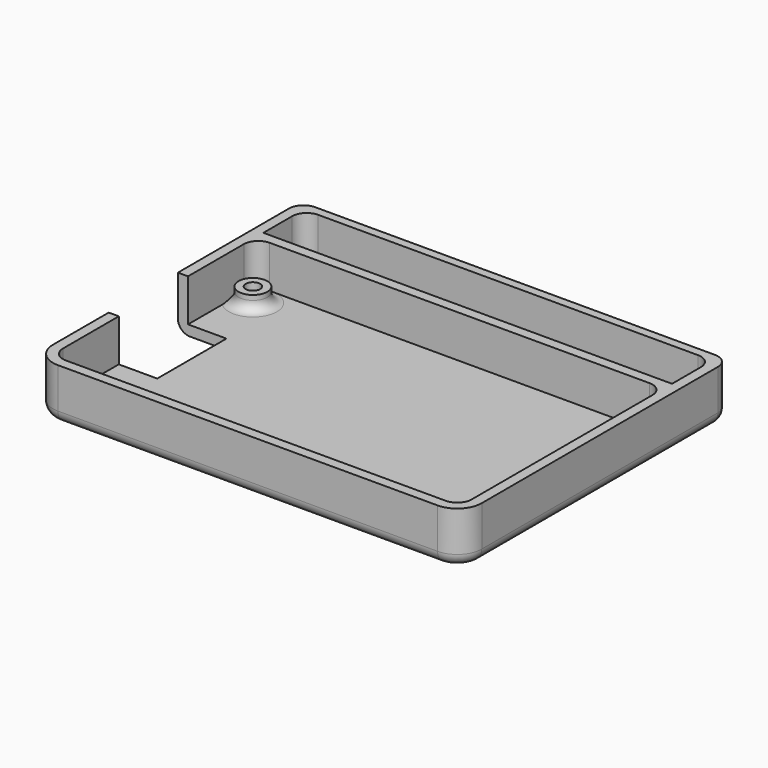
from build123d import *

# Parameters (mm, degrees)
F0_R         = 3
F0_R_2       = 1.5
F1_DEPTH     = 2.1
F2_DEPTH     = 10.9
F3_T1_DEPTH  = 61.4
F3_T3_DEPTH  = 83.2
F3_T5_DEPTH  = 35.15
F3_T7_DEPTH  = 20.75
F3_T9_DEPTH  = 79
F3_T12_ANGLE = 90
F3_T14_ANGLE = 90
F3_T16_ANGLE = 90
F3_T18_ANGLE = 90
F4_DEPTH     = 5.1


# Not quite as in the source:
# - a fillet or chamfer that OpenCascade refuses, or shapes differently, is made with other operations: its cross-section is extruded or revolved along the edge and cut away or added


with BuildPart() as f1:
    # F0 (on Top) → F1 (new body)
    with BuildSketch(Plane.XY):
        Polygon((34.5, 26.5), (-34.5, 26.5), (-34.5, 9), (-34.5, -9), (-34.5, -26.5), (34.5, -26.5), align=None)
        with BuildLine():
            add(Edge.make_bspline(
                [(-39.5, 28.6), (-36.7176169559, 28.6), (-36.7176169559, 33.85), (-36.7176169559, 39.1), (-39.5, 39.1)],
                knots=[3.1415926536, 3.1415926536, 3.1415926536, 4.7123889804, 4.7123889804, 6.2831853072, 6.2831853072, 6.2831853072], degree=2, weights=[1, 0.7071067812, 1, 0.7071067812, 1]))
            Line((-39.5, 28.6), (39.5, 28.6))
            Line((39.5, 28.6), (42.5, 28.6))
            Line((42.5, 28.6), (42.5, 36.1))
            ThreePointArc((42.5, 36.1), (41.6213203436, 38.2213203436), (39.5, 39.1))
            Line((39.5, 39.1), (0, 39.1))
            Line((0, 39.1), (-39.5, 39.1))
        make_face()
        with BuildLine():
            Line((-42.5, 9), (-42.5, 23.5))
            Line((-42.5, 23.5), (-42.5, 28.6))
            Line((-42.5, 28.6), (-42.5, 36.1))
            ThreePointArc((-42.5, 36.1), (-41.6213203436, 38.2213203436), (-39.5, 39.1))
            Line((-39.5, 39.1), (0, 39.1))
            Line((0, 39.1), (39.5, 39.1))
            ThreePointArc((39.5, 39.1), (41.6213203436, 38.2213203436), (42.5, 36.1))
            Line((42.5, 36.1), (42.5, 28.6))
            Line((42.5, 28.6), (42.5, 23.5))
            Line((42.5, 23.5), (42.5, -23.5))
            ThreePointArc((42.5, -23.5), (41.6213203436, -25.6213203436), (39.5, -26.5))
            Line((39.5, -26.5), (34.5, -26.5))
            Line((34.5, -26.5), (-34.5, -26.5))
            Line((-34.5, -26.5), (-39.5, -26.5))
            ThreePointArc((-39.5, -26.5), (-41.6213203436, -25.6213203436), (-42.5, -23.5))
            Line((-42.5, -23.5), (-42.5, -9))
            Line((-42.5, -9), (-44.6, -9))
            Line((-44.6, -9), (-44.6, -23.5))
            ThreePointArc((-44.6, -23.5), (-43.1062445841, -27.1062445841), (-39.5, -28.6))
            Line((-39.5, -28.6), (39.5, -28.6))
            ThreePointArc((39.5, -28.6), (43.1062445841, -27.1062445841), (44.6, -23.5))
            Line((44.6, -23.5), (44.6, 23.5))
            Line((44.6, 23.5), (44.6, 37.9))
            ThreePointArc((44.6, 37.9), (43.7213203436, 40.0213203436), (41.6, 40.9))
            Line((41.6, 40.9), (0, 40.9))
            Line((0, 40.9), (-41.6, 40.9))
            ThreePointArc((-41.6, 40.9), (-43.7213203436, 40.0213203436), (-44.6, 37.9))
            Line((-44.6, 37.9), (-44.6, 23.5))
            Line((-44.6, 23.5), (-44.6, 9))
            Line((-44.6, 9), (-42.5, 9))
        make_face()
        with BuildLine():
            Line((39.5, 26.5), (34.5, 26.5))
            Line((34.5, 26.5), (34.5, -26.5))
            Line((34.5, -26.5), (39.5, -26.5))
            ThreePointArc((39.5, -26.5), (41.6213203436, -25.6213203436), (42.5, -23.5))
            Line((42.5, -23.5), (42.5, 23.5))
            ThreePointArc((42.5, 23.5), (41.6213203436, 25.6213203436), (39.5, 26.5))
        make_face()
        with Locations((39, -21.5)):
            Circle(F0_R, mode=Mode.SUBTRACT)
        with Locations((39, 21.5)):
            Circle(F0_R, mode=Mode.SUBTRACT)
        with BuildLine():
            ThreePointArc((-42.5, 23.5), (-41.6213203436, 25.6213203436), (-39.5, 26.5))
            Line((-39.5, 26.5), (-34.5, 26.5))
            Line((-34.5, 26.5), (34.5, 26.5))
            Line((34.5, 26.5), (39.5, 26.5))
            ThreePointArc((39.5, 26.5), (41.6213203436, 25.6213203436), (42.5, 23.5))
            Line((42.5, 23.5), (42.5, 28.6))
            Line((42.5, 28.6), (39.5, 28.6))
            Line((39.5, 28.6), (-39.5, 28.6))
            Line((-39.5, 28.6), (-42.5, 28.6))
            Line((-42.5, 28.6), (-42.5, 23.5))
        make_face()
        with BuildLine():
            Line((-34.5, 26.5), (-39.5, 26.5))
            ThreePointArc((-39.5, 26.5), (-41.6213203436, 25.6213203436), (-42.5, 23.5))
            Line((-42.5, 23.5), (-42.5, 9))
            Line((-42.5, 9), (-34.5, 9))
            Line((-34.5, 9), (-34.5, 26.5))
        make_face()
        with Locations((-39, 21.5)):
            Circle(F0_R, mode=Mode.SUBTRACT)
        with BuildLine():
            Line((-34.5, -26.5), (-34.5, -9))
            Line((-34.5, -9), (-42.5, -9))
            Line((-42.5, -9), (-42.5, -23.5))
            ThreePointArc((-42.5, -23.5), (-41.6213203436, -25.6213203436), (-39.5, -26.5))
            Line((-39.5, -26.5), (-34.5, -26.5))
        make_face()
        with Locations((-39, -21.5)):
            Circle(F0_R, mode=Mode.SUBTRACT)
        with Locations((-39, 21.5)):
            Circle(F0_R)
        with Locations((-39, 21.5)):
            Circle(F0_R_2, mode=Mode.SUBTRACT)
        with Locations((-39, -21.5)):
            Circle(F0_R)
        with Locations((-39, -21.5)):
            Circle(F0_R_2, mode=Mode.SUBTRACT)
        with Locations((39, 21.5)):
            Circle(F0_R)
        with Locations((39, 21.5)):
            Circle(F0_R_2, mode=Mode.SUBTRACT)
        with Locations((39, -21.5)):
            Circle(F0_R)
        with Locations((39, -21.5)):
            Circle(F0_R_2, mode=Mode.SUBTRACT)
        with BuildLine():
            Line((-42.5, 36.1), (-42.5, 28.6))
            Line((-42.5, 28.6), (-39.5, 28.6))
            add(Edge.make_bspline(
                [(-39.5, 39.1), (-42.2823830441, 39.1), (-42.2823830441, 33.85), (-42.2823830441, 28.6), (-39.5, 28.6)],
                knots=[0, 0, 0, 1.5707963268, 1.5707963268, 3.1415926536, 3.1415926536, 3.1415926536], degree=2, weights=[1, 0.7071067812, 1, 0.7071067812, 1]))
            ThreePointArc((-39.5, 39.1), (-41.6213203436, 38.2213203436), (-42.5, 36.1))
        make_face()
    extrude(amount=F1_DEPTH)

    # F0 (on Top) → F2 (join)
    with BuildSketch(Plane.XY):
        with BuildLine():
            Line((-42.5, 9), (-42.5, 23.5))
            Line((-42.5, 23.5), (-42.5, 28.6))
            Line((-42.5, 28.6), (-42.5, 36.1))
            ThreePointArc((-42.5, 36.1), (-41.6213203436, 38.2213203436), (-39.5, 39.1))
            Line((-39.5, 39.1), (0, 39.1))
            Line((0, 39.1), (39.5, 39.1))
            ThreePointArc((39.5, 39.1), (41.6213203436, 38.2213203436), (42.5, 36.1))
            Line((42.5, 36.1), (42.5, 28.6))
            Line((42.5, 28.6), (42.5, 23.5))
            Line((42.5, 23.5), (42.5, -23.5))
            ThreePointArc((42.5, -23.5), (41.6213203436, -25.6213203436), (39.5, -26.5))
            Line((39.5, -26.5), (34.5, -26.5))
            Line((34.5, -26.5), (-34.5, -26.5))
            Line((-34.5, -26.5), (-39.5, -26.5))
            ThreePointArc((-39.5, -26.5), (-41.6213203436, -25.6213203436), (-42.5, -23.5))
            Line((-42.5, -23.5), (-42.5, -9))
            Line((-42.5, -9), (-44.6, -9))
            Line((-44.6, -9), (-44.6, -23.5))
            ThreePointArc((-44.6, -23.5), (-43.1062445841, -27.1062445841), (-39.5, -28.6))
            Line((-39.5, -28.6), (39.5, -28.6))
            ThreePointArc((39.5, -28.6), (43.1062445841, -27.1062445841), (44.6, -23.5))
            Line((44.6, -23.5), (44.6, 23.5))
            Line((44.6, 23.5), (44.6, 37.9))
            ThreePointArc((44.6, 37.9), (43.7213203436, 40.0213203436), (41.6, 40.9))
            Line((41.6, 40.9), (0, 40.9))
            Line((0, 40.9), (-41.6, 40.9))
            ThreePointArc((-41.6, 40.9), (-43.7213203436, 40.0213203436), (-44.6, 37.9))
            Line((-44.6, 37.9), (-44.6, 23.5))
            Line((-44.6, 23.5), (-44.6, 9))
            Line((-44.6, 9), (-42.5, 9))
        make_face()
        with BuildLine():
            ThreePointArc((-42.5, 23.5), (-41.6213203436, 25.6213203436), (-39.5, 26.5))
            Line((-39.5, 26.5), (-34.5, 26.5))
            Line((-34.5, 26.5), (34.5, 26.5))
            Line((34.5, 26.5), (39.5, 26.5))
            ThreePointArc((39.5, 26.5), (41.6213203436, 25.6213203436), (42.5, 23.5))
            Line((42.5, 23.5), (42.5, 28.6))
            Line((42.5, 28.6), (39.5, 28.6))
            Line((39.5, 28.6), (-39.5, 28.6))
            Line((-39.5, 28.6), (-42.5, 28.6))
            Line((-42.5, 28.6), (-42.5, 23.5))
        make_face()
    extrude(amount=F2_DEPTH)

    # F3: fillet of radius 2.5 on 9 edges, made by hand

    # F3_s2 → F3_t1 (cut)
    with BuildSketch(Plane.XZ.offset(-37.9)):
        with BuildLine():
            ThreePointArc((42.1, 0), (43.867766953, 0.732233047), (44.6, 2.5))
            Line((44.6, 2.5), (44.6, 0))
            Line((44.6, 0), (42.1, 0))
        make_face()
    extrude(amount=F3_T1_DEPTH, mode=Mode.SUBTRACT)

    # F3_s4 → F3_t3 (cut)
    with BuildSketch(Plane.YZ.offset(-41.6)):
        with BuildLine():
            ThreePointArc((38.4, 0), (40.167766953, 0.732233047), (40.9, 2.5))
            Line((40.9, 2.5), (40.9, 0))
            Line((40.9, 0), (38.4, 0))
        make_face()
    extrude(amount=F3_T3_DEPTH, mode=Mode.SUBTRACT)

    # F3_s6 → F3_t5 (cut)
    with BuildSketch(Plane.XZ.offset(-37.9)):
        with BuildLine():
            ThreePointArc((-42.1, 0), (-43.867766953, 0.732233047), (-44.6, 2.5))
            Line((-44.6, 2.5), (-44.6, 0))
            Line((-44.6, 0), (-42.1, 0))
        make_face()
    extrude(amount=F3_T5_DEPTH, mode=Mode.SUBTRACT)

    # F3_s8 → F3_t7 (cut)
    with BuildSketch(Plane.XZ.offset(2.75)):
        with BuildLine():
            ThreePointArc((-42.1, 0), (-43.867766953, 0.732233047), (-44.6, 2.5))
            Line((-44.6, 2.5), (-44.6, 0))
            Line((-44.6, 0), (-42.1, 0))
        make_face()
    extrude(amount=F3_T7_DEPTH, mode=Mode.SUBTRACT)

    # F3_s10 → F3_t9 (cut)
    with BuildSketch(Plane.YZ.offset(-39.5)):
        with BuildLine():
            ThreePointArc((-26.1, 0), (-27.867766953, 0.732233047), (-28.6, 2.5))
            Line((-28.6, 2.5), (-28.6, 0))
            Line((-28.6, 0), (-26.1, 0))
        make_face()
    extrude(amount=F3_T9_DEPTH, mode=Mode.SUBTRACT)

    # F3_s11 → F3_t12 (revolve, cut)
    with BuildSketch(Plane.YZ.offset(-41.6)):
        with BuildLine():
            ThreePointArc((40.9, 2.5), (40.167766953, 0.732233047), (38.4, 0))
            Line((38.4, 0), (40.9, 0))
            Line((40.9, 0), (40.9, 2.5))
        make_face()
    revolve(axis=Axis((-41.6, 37.9, 0), (0, 0, 1)), revolution_arc=F3_T12_ANGLE, mode=Mode.SUBTRACT)

    # F3_s13 → F3_t14 (revolve, cut)
    with BuildSketch(Plane.XZ.offset(23.5)):
        with BuildLine():
            ThreePointArc((-42.1, 0), (-43.867766953, 0.732233047), (-44.6, 2.5))
            Line((-44.6, 2.5), (-44.6, 0))
            Line((-44.6, 0), (-42.1, 0))
        make_face()
    revolve(axis=Axis((-39.5, -23.5, 0), (0, 0, 1)), revolution_arc=F3_T14_ANGLE, mode=Mode.SUBTRACT)

    # F3_s15 → F3_t16 (revolve, cut)
    with BuildSketch(Plane.YZ.offset(39.5)):
        with BuildLine():
            ThreePointArc((-26.1, 0), (-27.867766953, 0.732233047), (-28.6, 2.5))
            Line((-28.6, 2.5), (-28.6, 0))
            Line((-28.6, 0), (-26.1, 0))
        make_face()
    revolve(axis=Axis((39.5, -23.5, 0), (0, 0, 1)), revolution_arc=F3_T16_ANGLE, mode=Mode.SUBTRACT)

    # F3_s17 → F3_t18 (revolve, cut)
    with BuildSketch(Plane.XZ.offset(-37.9)):
        with BuildLine():
            ThreePointArc((42.1, 0), (43.867766953, 0.732233047), (44.6, 2.5))
            Line((44.6, 2.5), (44.6, 0))
            Line((44.6, 0), (42.1, 0))
        make_face()
    revolve(axis=Axis((41.6, 37.9, 0), (0, 0, 1)), revolution_arc=F3_T18_ANGLE, mode=Mode.SUBTRACT)

    # F0 (on Top) → F4 (join)
    with BuildSketch(Plane.XY):
        with Locations((-39, 21.5)):
            Circle(F0_R)
        with Locations((-39, 21.5)):
            Circle(F0_R_2, mode=Mode.SUBTRACT)
        with Locations((39, 21.5)):
            Circle(F0_R)
        with Locations((39, 21.5)):
            Circle(F0_R_2, mode=Mode.SUBTRACT)
        with Locations((39, -21.5)):
            Circle(F0_R)
        with Locations((39, -21.5)):
            Circle(F0_R_2, mode=Mode.SUBTRACT)
        with Locations((-39, -21.5)):
            Circle(F0_R)
        with Locations((-39, -21.5)):
            Circle(F0_R_2, mode=Mode.SUBTRACT)
    extrude(amount=F4_DEPTH)

    # F5: fillet of radius 2 on 4 edges, made by hand

    # F5_s1 → F5_t2 (revolve)
    with BuildSketch(Plane.XZ.offset(-21.5)):
        with BuildLine():
            ThreePointArc((-34, 2.1), (-35.4142135624, 2.6857864376), (-36, 4.1))
            Line((-36, 4.1), (-36, 2.1))
            Line((-36, 2.1), (-34, 2.1))
        make_face()
    revolve(axis=Axis((-39, 21.5, 2.1), (0, 0, -1)))

    # F5_s3 → F5_t4 (revolve)
    with BuildSketch(Plane.XZ.offset(-21.5)):
        with BuildLine():
            ThreePointArc((44, 2.1), (42.5857864376, 2.6857864376), (42, 4.1))
            Line((42, 4.1), (42, 2.1))
            Line((42, 2.1), (44, 2.1))
        make_face()
    revolve(axis=Axis((39, 21.5, 2.1), (0, 0, -1)))

    # F5_s5 → F5_t6 (revolve)
    with BuildSketch(Plane.XZ.offset(21.5)):
        with BuildLine():
            ThreePointArc((44, 2.1), (42.5857864376, 2.6857864376), (42, 4.1))
            Line((42, 4.1), (42, 2.1))
            Line((42, 2.1), (44, 2.1))
        make_face()
    revolve(axis=Axis((39, -21.5, 2.1), (0, 0, -1)))

    # F5_s7 → F5_t8 (revolve)
    with BuildSketch(Plane.XZ.offset(21.5)):
        with BuildLine():
            ThreePointArc((-34, 2.1), (-35.4142135624, 2.6857864376), (-36, 4.1))
            Line((-36, 4.1), (-36, 2.1))
            Line((-36, 2.1), (-34, 2.1))
        make_face()
    revolve(axis=Axis((-39, -21.5, 2.1), (0, 0, -1)))


solid = f1.part
